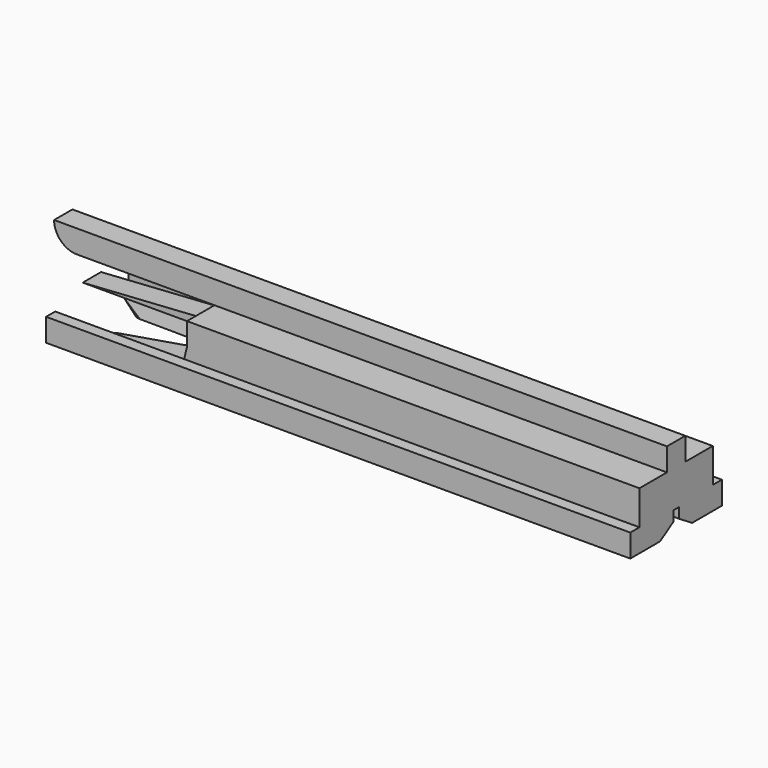
from build123d import *

# Parameters (mm, degrees)
F0_W      = 30
F0_H      = 5
F1_DEPTH  = 8
F4_DEPTH  = 51.001
F5_DEPTH  = 5.001
F6_W      = 1
F6_H      = 2
F7_DEPTH  = 51
F8_W      = 2
F8_H      = 0.75
F9_DEPTH  = 11.5
F11_DEPTH = 6.001
F12_W     = 39.5
F12_H     = 2
F12_W_2   = 14
F13_DEPTH = 2
F14_R     = 1.99999


# Not quite as in the source:
# - a fillet or chamfer is up to 0.001 mm smaller than in the source, because OpenCascade refuses the exact size


with BuildPart() as f1:
    # F0 (on Front) → F1 (new body)
    with BuildSketch(Plane.XZ):
        Polygon((0, 0), (0, 5), (-9.5, 5), (-9.5, 3), (-10, 1), (-21, 0), align=None)
        with Locations((15, 2.5)):
            Rectangle(F0_W, F0_H)
    extrude(amount=F1_DEPTH)

    # F3 (on face) → F4 (cut, through all)
    with BuildSketch(Plane.YZ.offset(30)):
        Polygon((-3.7, 1.8), (-4.3, 1.8), (-4.3, 0.9114285714), (-4, 1.1), (-3.7, 0.9114285714), align=None)
        Polygon((-4.3, 0), (-4.3, 0.9114285714), (-5.75, 0), align=None)
        Polygon((-2.25, 0), (-3.7, 0.9114285714), (-3.7, 0), align=None)
        Polygon((-4, 1.1), (-4.3, 0.9114285714), (-4.3, 0), (-3.7, 0), (-3.7, 0.9114285714), align=None)
    extrude(amount=-F4_DEPTH, mode=Mode.SUBTRACT)

    # F2 (on face) → F5 (cut, through all)
    with BuildSketch(Plane(origin=(0, 0, 0), x_dir=(1, 0, 0), z_dir=(0, 0, -1))):
        Polygon((-16, 4), (-21, 7.5), (-21, 0.5), align=None)
    extrude(amount=-F5_DEPTH, mode=Mode.SUBTRACT)

    # F6 (on face) → F7 (join, through all)
    with BuildSketch(Plane.YZ.offset(30)):
        with Locations((-8.5, 1)):
            Rectangle(F6_W, F6_H)
        with Locations((0.5, 1)):
            Rectangle(F6_W, F6_H)
    extrude(amount=-F7_DEPTH)

    # F8 (on face) → F9 (join)
    with BuildSketch(Plane(origin=(-9.5, 0, 0), x_dir=(0, -1, 0), z_dir=(-1, 0, 0))):
        with Locations((4, 3.375)):
            Rectangle(F8_W, F8_H)
    extrude(amount=F9_DEPTH)

    # F10 (on face) → F11 (cut, through all)
    with BuildSketch(Plane.XZ.offset(5)):
        Polygon((-21, 3.75), (-21, 3), (-9.5, 3.75), align=None)
    extrude(amount=-F11_DEPTH, mode=Mode.SUBTRACT)

    # F12 (on face) → F13 (join)
    with BuildSketch(Plane.XY.offset(5)):
        with Locations((10.25, -4)):
            Rectangle(F12_W, F12_H)
        with Locations((-16.5, -4)):
            Rectangle(F12_W_2, F12_H)
    extrude(amount=F13_DEPTH)

    # F14 (radius 2 in the source; OpenCascade refuses exactly that, so slightly less here)
    f14_edges = [f1.edges().sort_by_distance(p)[0] for p in [
        (-23.5, -4, 5),
    ]]
    fillet(f14_edges, radius=F14_R)


solid = f1.part
